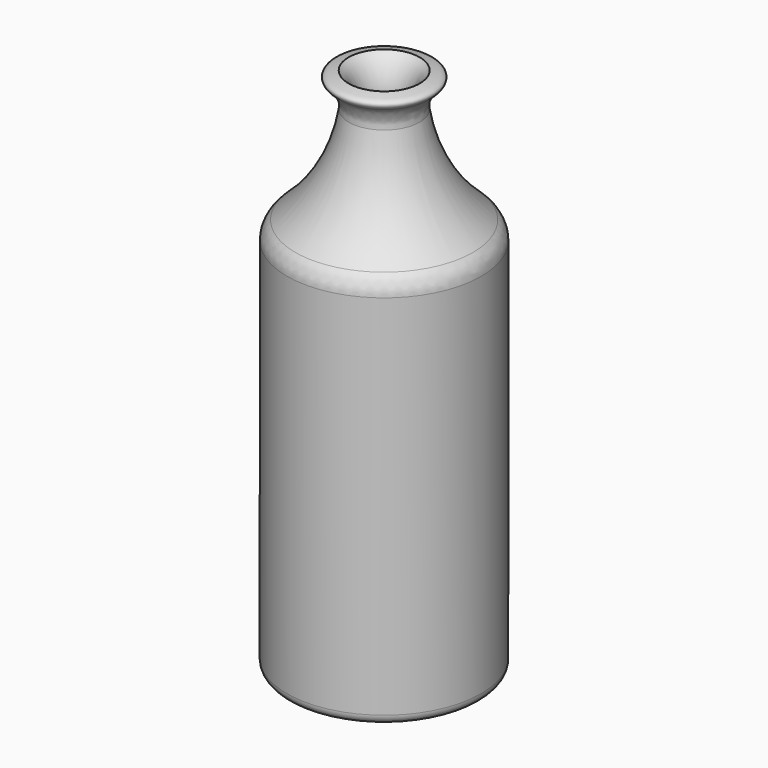
from build123d import *

# Parameters (mm, degrees)
F2_R = 5
F3_T = 3


# Not quite as in the source:
# - a shell that OpenCascade refuses in one call is made with other operations: the cavity is built on its own and cut out


with BuildPart() as f1:
    # F0 (on Front) → F1 (revolve)
    with BuildSketch(Plane.XZ):
        with BuildLine():
            Line((0.0303446585, 43.9893868108), (0, -60))
            Line((0, -60), (18, -60))
            ThreePointArc((18, -60), (19.4142135624, -59.4142135624), (20, -58))
            Line((20, -58), (20, 20))
            ThreePointArc((20, 20), (10.699829352, 31.0439112631), (7, 45))
            add(Edge.make_bspline(
                [(7, 45), (5.0981917384, 44.3288351313), (2.5656114194, 43.9919770233), (0.0303446585, 43.9893868108)],
                knots=[0.7335604777, 0.7335604777, 0.7335604777, 0.7335604777, 0.8662634951, 0.8662634951, 0.8662634951, 0.8662634951], degree=3))
        make_face()
        with BuildLine():
            Line((0.0317348174, 48.7533809147), (0.0303446585, 43.9893868108))
            add(Edge.make_bspline(
                [(7, 45), (5.0981917384, 44.3288351313), (2.5656114194, 43.9919770233), (0.0303446585, 43.9893868108)],
                knots=[0.7335604777, 0.7335604777, 0.7335604777, 0.7335604777, 0.8662634951, 0.8662634951, 0.8662634951, 0.8662634951], degree=3))
            add(Edge.make_bspline(
                [(0.0317348174, 48.7533809147), (4.7629433155, 48.7522243079), (12.4211351263, 48.5438301873), (9.0166847824, 45.7117058036), (7, 45)],
                knots=[0.3671333927, 0.3671333927, 0.3671333927, 0.3671333927, 0.5928416886, 0.7335604777, 0.7335604777, 0.7335604777, 0.7335604777], degree=3))
        make_face()
        with BuildLine():
            add(Edge.make_bspline(
                [(0.0303446585, 43.9893868108), (-2.5246666918, 43.9867764257), (-5.0824064908, 44.3236607489), (-7, 45)],
                knots=[0.8662634951, 0.8662634951, 0.8662634951, 0.8662634951, 1, 1, 1, 1], degree=3))
            Line((0.0303446585, 43.9893868108), (0.0317348174, 48.7533809147))
            add(Edge.make_bspline(
                [(-7, 45), (-9.0177096511, 45.7116504242), (-12.4328083134, 48.5488604685), (-4.7142790246, 48.7545411409), (0.0317348174, 48.7533809147)],
                knots=[0, 0, 0, 0, 0.1407187891, 0.3671333927, 0.3671333927, 0.3671333927, 0.3671333927], degree=3))
        make_face()
    revolve(axis=Axis((0.0158674087, 0, -5.6233095426), (-0.0002918053, 0, -0.9999999574)))

    # F2
    f2_edges = [f1.edges().sort_by_distance(p)[0] for p in [
        (-19.953308, 0, 20.011659),
        (-6.93872, 0, 45.004067),
    ]]
    fillet(f2_edges, radius=F2_R)

    # F3: shell of thickness 3, made by hand


with BuildPart() as f3_core1:
    # F3_t2: copy of F1
    add(f1.part)

    # the walls: a layer under each face that stays
    f3_faces = [f3_core1.faces().sort_by_distance(p)[0] for p in [
        (-19.9767604628, 0, -20.1738934498),
        (-19.5052168736, 0, 19.7095019558),
        (-10.9686231738, 0, 30.4472386816),
        (-8.9999984673, 0, -59.9947475043),
        (-7.5836491668, 0, 44.0565358923),
    ]]
    thicken(f3_faces, amount=-F3_T, mode=Mode.SUBTRACT)


with BuildPart() as f1_1:
    add(f1.part)

    # what is left inside the walls is the cavity
    f3_cavity = [f3_core1.part.solids().sort_by_distance(p)[0] for p in [
        (-16.953728, 0, -32.113807),
    ]]
    add(f3_cavity, mode=Mode.SUBTRACT)


solid = f1_1.part
